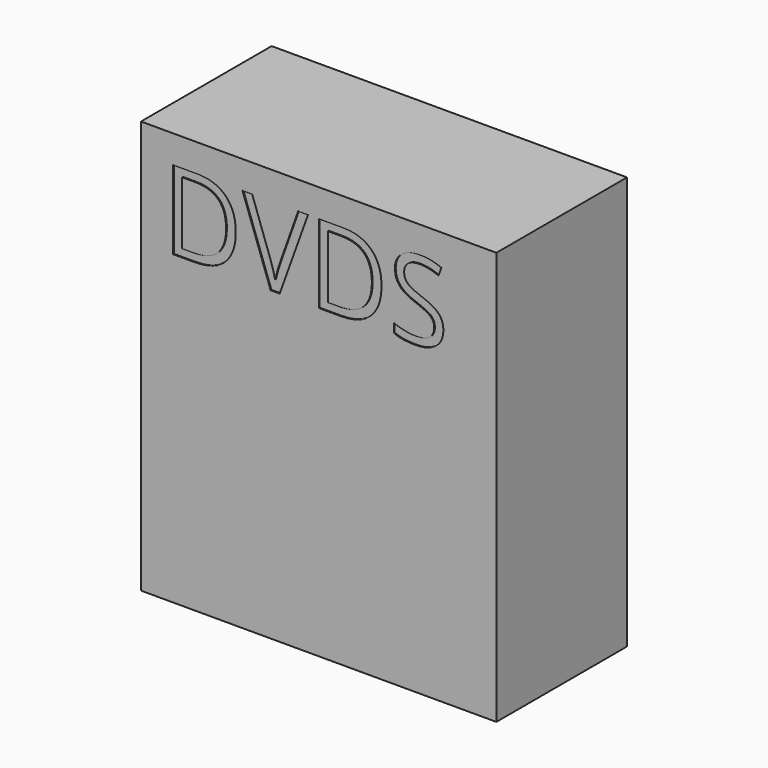
from build123d import *

# Parameters (mm, degrees)
F0_W         = 370
F0_H         = 170
F1_DEPTH     = 430
F2_TEXT_SIZE = 114.5712617371
F3_DEPTH     = 1


# Not quite as in the source:
# - Text() gives the source's letters only with a copy of the font that has no kerning and outlines rounded to 1/6400 em; it was checked with that copy


with BuildPart() as f1:
    # F0 (on Top) → F1 (new body)
    with BuildSketch(Plane.XY):
        Rectangle(F0_W, F0_H)
    extrude(amount=F1_DEPTH)

    # F2 (on face) → F3 (cut)
    with BuildSketch(Plane.XZ.offset(85)):
        with Locations((-162.8449112177, 319.1946148872)):
            Text('DVDS', F2_TEXT_SIZE, font='Open Sans', text_align=(TextAlign.LEFT, TextAlign.BOTTOM))
    extrude(amount=-F3_DEPTH, mode=Mode.SUBTRACT)


solid = f1.part
